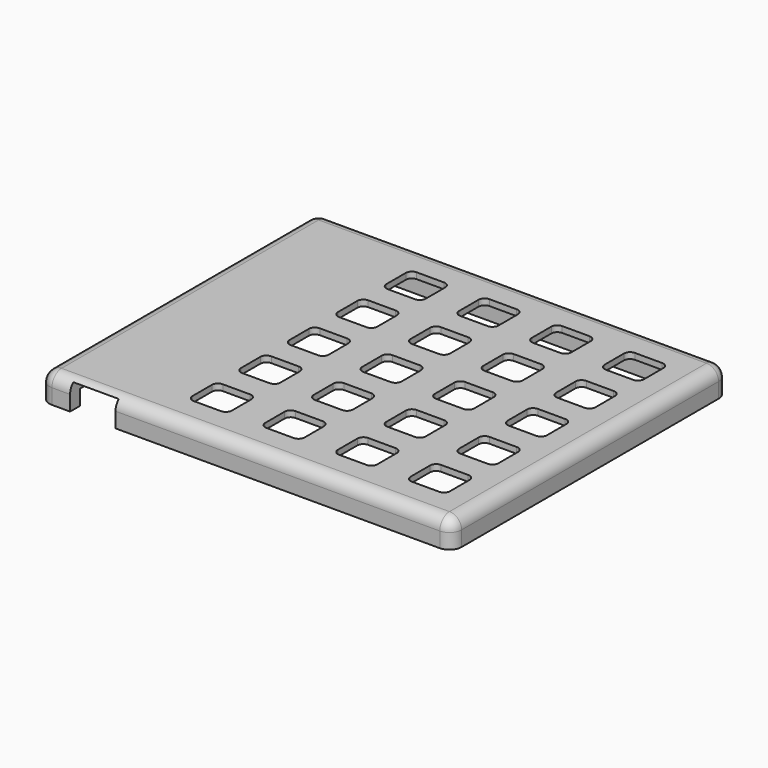
from build123d import *

# Parameters (mm, degrees)
F0_W          = 107.95
F0_H          = 90.4875
F1_DEPTH      = 7.14375
F2_W          = 101.6
F2_H          = 81.75625
F3_DEPTH      = 3.96875
F4_W          = 15.08125
F4_H          = 14.2875
F4_W_2        = 11.90625
F4_H_2        = 11.1125
F4_W_3        = 1.5875
F4_H_3        = 1.5875
F5_DEPTH      = 1.5875
F8_DEPTH      = 25.4
F9_W          = 11.90625
F9_H          = 6.35
F10_DEPTH     = 4.7625
F11_T1_DEPTH  = 101.6
F11_T3_DEPTH  = 84.1375
F11_T5_DEPTH  = 11.90625
F11_S9_W      = 3.175
F11_S9_H      = 3.175
F11_T10_DEPTH = 3.175
F11_S15_W     = 3.175
F11_S15_H     = 3.175
F11_T16_DEPTH = 3.175
F11_S21_W     = 3.175
F11_S21_H     = 3.175
F11_T22_DEPTH = 3.175
F11_S27_W     = 3.175
F11_S27_H     = 3.175
F11_T28_DEPTH = 3.175
F13_W         = 4.92252
F13_H         = 5.31749
F14_DEPTH     = 3.96875


# Not quite as in the source:
# - a fillet or chamfer that OpenCascade refuses, or shapes differently, is made with other operations: its cross-section is extruded or revolved along the edge and cut away or added


with BuildPart() as f1:
    # F0 (on Top) → F1 (new body)
    with BuildSketch(Plane.XY):
        Rectangle(F0_W, F0_H)
    extrude(amount=F1_DEPTH)

    # F2 (on face) → F3 (cut)
    with BuildSketch(Plane(origin=(0, 0, 0), x_dir=(1, 0, 0), z_dir=(0, 0, -1))):
        with Locations((0, 1.190625)):
            Rectangle(F2_W, F2_H)
    extrude(amount=-F3_DEPTH, mode=Mode.SUBTRACT)

    # F4 (on face) → F5 (cut)
    with BuildSketch(Plane(origin=(0, 0, 3.96875), x_dir=(1, 0, 0), z_dir=(0, 0, -1))):
        Polygon((-24.60625, 38.89375), (-24.60625, 34.7782671452), (-24.60625, 24.60625), (-9.525, 24.60625), (-9.525, 38.89375), align=None)
        Polygon((-23.01875, 26.19375), (-23.01875, 34.7782671452), (-23.01875, 37.30625), (-11.1125, 37.30625), (-11.1125, 26.19375), align=None, mode=Mode.SUBTRACT)
        with Locations((1.984375, 31.75)):
            Rectangle(F4_W, F4_H)
        with Locations((1.984375, 31.75)):
            Rectangle(F4_W_2, F4_H_2, mode=Mode.SUBTRACT)
        with Locations((21.034375, 31.75)):
            Rectangle(F4_W, F4_H)
        with Locations((21.034375, 31.75)):
            Rectangle(F4_W_2, F4_H_2, mode=Mode.SUBTRACT)
        with Locations((40.084375, 15.875)):
            Rectangle(F4_W, F4_H)
        with Locations((40.084375, 15.875)):
            Rectangle(F4_W_2, F4_H_2, mode=Mode.SUBTRACT)
        with Locations((21.034375, 15.875)):
            Rectangle(F4_W, F4_H)
        with Locations((21.034375, 15.875)):
            Rectangle(F4_W_2, F4_H_2, mode=Mode.SUBTRACT)
        with Locations((1.984375, 15.875)):
            Rectangle(F4_W, F4_H)
        with Locations((1.984375, 15.875)):
            Rectangle(F4_W_2, F4_H_2, mode=Mode.SUBTRACT)
        with Locations((-17.065625, 15.875)):
            Rectangle(F4_W, F4_H)
        with Locations((-17.065625, 15.875)):
            Rectangle(F4_W_2, F4_H_2, mode=Mode.SUBTRACT)
        with Locations((-17.065625, 0)):
            Rectangle(F4_W, F4_H)
        with Locations((-17.065625, 0)):
            Rectangle(F4_W_2, F4_H_2, mode=Mode.SUBTRACT)
        with Locations((1.984375, 0)):
            Rectangle(F4_W, F4_H)
        with Locations((1.984375, 0)):
            Rectangle(F4_W_2, F4_H_2, mode=Mode.SUBTRACT)
        with Locations((21.034375, 0)):
            Rectangle(F4_W, F4_H)
        with Locations((21.034375, 0)):
            Rectangle(F4_W_2, F4_H_2, mode=Mode.SUBTRACT)
        with Locations((40.084375, 0)):
            Rectangle(F4_W, F4_H)
        with Locations((40.084375, 0)):
            Rectangle(F4_W_2, F4_H_2, mode=Mode.SUBTRACT)
        with Locations((-17.065625, -15.875)):
            Rectangle(F4_W, F4_H)
        with Locations((-17.065625, -15.875)):
            Rectangle(F4_W_2, F4_H_2, mode=Mode.SUBTRACT)
        with Locations((1.984375, -15.875)):
            Rectangle(F4_W, F4_H)
        with Locations((1.984375, -15.875)):
            Rectangle(F4_W_2, F4_H_2, mode=Mode.SUBTRACT)
        with Locations((21.034375, -15.875)):
            Rectangle(F4_W, F4_H)
        with Locations((21.034375, -15.875)):
            Rectangle(F4_W_2, F4_H_2, mode=Mode.SUBTRACT)
        with Locations((40.084375, -15.875)):
            Rectangle(F4_W, F4_H)
        with Locations((40.084375, -15.875)):
            Rectangle(F4_W_2, F4_H_2, mode=Mode.SUBTRACT)
        Polygon((32.54375, -38.89375), (41.1446839571, -38.89375), (47.625, -38.89375), (47.625, -24.60625), (32.54375, -24.60625), align=None)
        Polygon((46.0375, -37.30625), (41.1446839571, -37.30625), (34.13125, -37.30625), (34.13125, -26.19375), (46.0375, -26.19375), align=None, mode=Mode.SUBTRACT)
        with Locations((21.034375, -31.75)):
            Rectangle(F4_W, F4_H)
        with Locations((21.034375, -31.75)):
            Rectangle(F4_W_2, F4_H_2, mode=Mode.SUBTRACT)
        with Locations((1.984375, -31.75)):
            Rectangle(F4_W, F4_H)
        with Locations((1.984375, -31.75)):
            Rectangle(F4_W_2, F4_H_2, mode=Mode.SUBTRACT)
        with Locations((-17.065625, -31.75)):
            Rectangle(F4_W, F4_H)
        with Locations((-17.065625, -31.75)):
            Rectangle(F4_W_2, F4_H_2, mode=Mode.SUBTRACT)
        Polygon((46.0375, 37.30625), (46.0375, 38.89375), (32.54375, 38.89375), (32.54375, 24.60625), (47.625, 24.60625), (47.625, 37.30625), align=None)
        with Locations((40.084375, 31.75)):
            Rectangle(F4_W_2, F4_H_2, mode=Mode.SUBTRACT)
        Polygon((-23.01875, 37.30625), (-23.01875, 34.7782671452), (-23.01875, 26.19375), (-11.1125, 26.19375), (-11.1125, 37.30625), align=None)
        with Locations((1.984375, 31.75)):
            Rectangle(F4_W_2, F4_H_2)
        with Locations((21.034375, 31.75)):
            Rectangle(F4_W_2, F4_H_2)
        with Locations((40.084375, 31.75)):
            Rectangle(F4_W_2, F4_H_2)
        with Locations((40.084375, 15.875)):
            Rectangle(F4_W_2, F4_H_2)
        with Locations((21.034375, 15.875)):
            Rectangle(F4_W_2, F4_H_2)
        with Locations((1.984375, 15.875)):
            Rectangle(F4_W_2, F4_H_2)
        with Locations((-17.065625, 15.875)):
            Rectangle(F4_W_2, F4_H_2)
        with Locations((-17.065625, 0)):
            Rectangle(F4_W_2, F4_H_2)
        with Locations((1.984375, 0)):
            Rectangle(F4_W_2, F4_H_2)
        with Locations((21.034375, 0)):
            Rectangle(F4_W_2, F4_H_2)
        with Locations((40.084375, 0)):
            Rectangle(F4_W_2, F4_H_2)
        with Locations((-17.065625, -15.875)):
            Rectangle(F4_W_2, F4_H_2)
        with Locations((1.984375, -15.875)):
            Rectangle(F4_W_2, F4_H_2)
        with Locations((21.034375, -15.875)):
            Rectangle(F4_W_2, F4_H_2)
        with Locations((40.084375, -15.875)):
            Rectangle(F4_W_2, F4_H_2)
        Polygon((34.13125, -37.30625), (41.1446839571, -37.30625), (46.0375, -37.30625), (46.0375, -26.19375), (34.13125, -26.19375), align=None)
        with Locations((21.034375, -31.75)):
            Rectangle(F4_W_2, F4_H_2)
        with Locations((1.984375, -31.75)):
            Rectangle(F4_W_2, F4_H_2)
        with Locations((-17.065625, -31.75)):
            Rectangle(F4_W_2, F4_H_2)
        with Locations((46.83125, 38.1)):
            Rectangle(F4_W_3, F4_H_3)
    extrude(amount=-F5_DEPTH, mode=Mode.SUBTRACT)

    # F7 (on face) → F8 (cut)
    with BuildSketch(Plane.XY.offset(7.14375)):
        with BuildLine():
            Line((43.65625, -26.9875), (36.5125, -26.9875))
            ThreePointArc((36.5125, -26.9875), (35.3899679849, -27.4524679849), (34.925, -28.575))
            Line((34.925, -28.575), (34.925, -34.925))
            ThreePointArc((34.925, -34.925), (35.3899679849, -36.0475320151), (36.5125, -36.5125))
            Line((36.5125, -36.5125), (43.65625, -36.5125))
            ThreePointArc((43.65625, -36.5125), (44.7787820151, -36.0475320151), (45.24375, -34.925))
            Line((45.24375, -34.925), (45.24375, -28.575))
            ThreePointArc((45.24375, -28.575), (44.7787820151, -27.4524679849), (43.65625, -26.9875))
        make_face()
        with BuildLine():
            Line((43.65625, -11.1125), (36.5125, -11.1125))
            ThreePointArc((36.5125, -11.1125), (35.3899679849, -11.5774679849), (34.925, -12.7))
            Line((34.925, -12.7), (34.925, -19.05))
            ThreePointArc((34.925, -19.05), (35.3899679849, -20.1725320151), (36.5125, -20.6375))
            Line((36.5125, -20.6375), (43.65625, -20.6375))
            ThreePointArc((43.65625, -20.6375), (44.7787820151, -20.1725320151), (45.24375, -19.05))
            Line((45.24375, -19.05), (45.24375, -12.7))
            ThreePointArc((45.24375, -12.7), (44.7787820151, -11.5774679849), (43.65625, -11.1125))
        make_face()
        with BuildLine():
            Line((24.60625, -11.1125), (17.4625, -11.1125))
            ThreePointArc((17.4625, -11.1125), (16.3399679849, -11.5774679849), (15.875, -12.7))
            Line((15.875, -12.7), (15.875, -19.05))
            ThreePointArc((15.875, -19.05), (16.3399679849, -20.1725320151), (17.4625, -20.6375))
            Line((17.4625, -20.6375), (24.60625, -20.6375))
            ThreePointArc((24.60625, -20.6375), (25.7287820151, -20.1725320151), (26.19375, -19.05))
            Line((26.19375, -19.05), (26.19375, -12.7))
            ThreePointArc((26.19375, -12.7), (25.7287820151, -11.5774679849), (24.60625, -11.1125))
        make_face()
        with BuildLine():
            Line((24.60625, -26.9875), (17.4625, -26.9875))
            ThreePointArc((17.4625, -26.9875), (16.3399679849, -27.4524679849), (15.875, -28.575))
            Line((15.875, -28.575), (15.875, -34.925))
            ThreePointArc((15.875, -34.925), (16.3399679849, -36.0475320151), (17.4625, -36.5125))
            Line((17.4625, -36.5125), (24.60625, -36.5125))
            ThreePointArc((24.60625, -36.5125), (25.7287820151, -36.0475320151), (26.19375, -34.925))
            Line((26.19375, -34.925), (26.19375, -28.575))
            ThreePointArc((26.19375, -28.575), (25.7287820151, -27.4524679849), (24.60625, -26.9875))
        make_face()
        with BuildLine():
            Line((5.55625, -26.9875), (-1.5875, -26.9875))
            ThreePointArc((-1.5875, -26.9875), (-2.7100320151, -27.4524679849), (-3.175, -28.575))
            Line((-3.175, -28.575), (-3.175, -34.925))
            ThreePointArc((-3.175, -34.925), (-2.7100320151, -36.0475320151), (-1.5875, -36.5125))
            Line((-1.5875, -36.5125), (5.55625, -36.5125))
            ThreePointArc((5.55625, -36.5125), (6.6787820151, -36.0475320151), (7.14375, -34.925))
            Line((7.14375, -34.925), (7.14375, -28.575))
            ThreePointArc((7.14375, -28.575), (6.6787820151, -27.4524679849), (5.55625, -26.9875))
        make_face()
        with BuildLine():
            Line((5.55625, -11.1125), (-1.5875, -11.1125))
            ThreePointArc((-1.5875, -11.1125), (-2.7100320151, -11.5774679849), (-3.175, -12.7))
            Line((-3.175, -12.7), (-3.175, -19.05))
            ThreePointArc((-3.175, -19.05), (-2.7100320151, -20.1725320151), (-1.5875, -20.6375))
            Line((-1.5875, -20.6375), (5.55625, -20.6375))
            ThreePointArc((5.55625, -20.6375), (6.6787820151, -20.1725320151), (7.14375, -19.05))
            Line((7.14375, -19.05), (7.14375, -12.7))
            ThreePointArc((7.14375, -12.7), (6.6787820151, -11.5774679849), (5.55625, -11.1125))
        make_face()
        with BuildLine():
            Line((-13.49375, -11.1125), (-20.6375, -11.1125))
            ThreePointArc((-20.6375, -11.1125), (-21.7600320151, -11.5774679849), (-22.225, -12.7))
            Line((-22.225, -12.7), (-22.225, -19.05))
            ThreePointArc((-22.225, -19.05), (-21.7600320151, -20.1725320151), (-20.6375, -20.6375))
            Line((-20.6375, -20.6375), (-13.49375, -20.6375))
            ThreePointArc((-13.49375, -20.6375), (-12.3712179849, -20.1725320151), (-11.90625, -19.05))
            Line((-11.90625, -19.05), (-11.90625, -12.7))
            ThreePointArc((-11.90625, -12.7), (-12.3712179849, -11.5774679849), (-13.49375, -11.1125))
        make_face()
        with BuildLine():
            Line((-13.49375, -26.9875), (-20.6375, -26.9875))
            ThreePointArc((-20.6375, -26.9875), (-21.7600320151, -27.4524679849), (-22.225, -28.575))
            Line((-22.225, -28.575), (-22.225, -34.925))
            ThreePointArc((-22.225, -34.925), (-21.7600320151, -36.0475320151), (-20.6375, -36.5125))
            Line((-20.6375, -36.5125), (-13.49375, -36.5125))
            ThreePointArc((-13.49375, -36.5125), (-12.3712179849, -36.0475320151), (-11.90625, -34.925))
            Line((-11.90625, -34.925), (-11.90625, -28.575))
            ThreePointArc((-11.90625, -28.575), (-12.3712179849, -27.4524679849), (-13.49375, -26.9875))
        make_face()
        with BuildLine():
            Line((-13.49375, 4.7625), (-20.6375, 4.7625))
            ThreePointArc((-20.6375, 4.7625), (-21.7600320151, 4.2975320151), (-22.225, 3.175))
            Line((-22.225, 3.175), (-22.225, -3.175))
            ThreePointArc((-22.225, -3.175), (-21.7600320151, -4.2975320151), (-20.6375, -4.7625))
            Line((-20.6375, -4.7625), (-13.49375, -4.7625))
            ThreePointArc((-13.49375, -4.7625), (-12.3712179849, -4.2975320151), (-11.90625, -3.175))
            Line((-11.90625, -3.175), (-11.90625, 3.175))
            ThreePointArc((-11.90625, 3.175), (-12.3712179849, 4.2975320151), (-13.49375, 4.7625))
        make_face()
        with BuildLine():
            Line((-13.49375, 20.6375), (-20.6375, 20.6375))
            ThreePointArc((-20.6375, 20.6375), (-21.7600320151, 20.1725320151), (-22.225, 19.05))
            Line((-22.225, 19.05), (-22.225, 12.7))
            ThreePointArc((-22.225, 12.7), (-21.7600320151, 11.5774679849), (-20.6375, 11.1125))
            Line((-20.6375, 11.1125), (-13.49375, 11.1125))
            ThreePointArc((-13.49375, 11.1125), (-12.3712179849, 11.5774679849), (-11.90625, 12.7))
            Line((-11.90625, 12.7), (-11.90625, 19.05))
            ThreePointArc((-11.90625, 19.05), (-12.3712179849, 20.1725320151), (-13.49375, 20.6375))
        make_face()
        with BuildLine():
            Line((-13.49375, 36.5125), (-20.6375, 36.5125))
            ThreePointArc((-20.6375, 36.5125), (-21.7600320151, 36.0475320151), (-22.225, 34.925))
            Line((-22.225, 34.925), (-22.225, 28.575))
            ThreePointArc((-22.225, 28.575), (-21.7600320151, 27.4524679849), (-20.6375, 26.9875))
            Line((-20.6375, 26.9875), (-13.49375, 26.9875))
            ThreePointArc((-13.49375, 26.9875), (-12.3712179849, 27.4524679849), (-11.90625, 28.575))
            Line((-11.90625, 28.575), (-11.90625, 34.925))
            ThreePointArc((-11.90625, 34.925), (-12.3712179849, 36.0475320151), (-13.49375, 36.5125))
        make_face()
        with BuildLine():
            Line((5.55625, 36.5125), (-1.5875, 36.5125))
            ThreePointArc((-1.5875, 36.5125), (-2.7100320151, 36.0475320151), (-3.175, 34.925))
            Line((-3.175, 34.925), (-3.175, 28.575))
            ThreePointArc((-3.175, 28.575), (-2.7100320151, 27.4524679849), (-1.5875, 26.9875))
            Line((-1.5875, 26.9875), (5.55625, 26.9875))
            ThreePointArc((5.55625, 26.9875), (6.6787820151, 27.4524679849), (7.14375, 28.575))
            Line((7.14375, 28.575), (7.14375, 34.925))
            ThreePointArc((7.14375, 34.925), (6.6787820151, 36.0475320151), (5.55625, 36.5125))
        make_face()
        with BuildLine():
            Line((24.60625, 36.5125), (17.4625, 36.5125))
            ThreePointArc((17.4625, 36.5125), (16.3399679849, 36.0475320151), (15.875, 34.925))
            Line((15.875, 34.925), (15.875, 28.575))
            ThreePointArc((15.875, 28.575), (16.3399679849, 27.4524679849), (17.4625, 26.9875))
            Line((17.4625, 26.9875), (24.60625, 26.9875))
            ThreePointArc((24.60625, 26.9875), (25.7287820151, 27.4524679849), (26.19375, 28.575))
            Line((26.19375, 28.575), (26.19375, 34.925))
            ThreePointArc((26.19375, 34.925), (25.7287820151, 36.0475320151), (24.60625, 36.5125))
        make_face()
        with BuildLine():
            Line((43.65625, 36.5125), (36.5125, 36.5125))
            ThreePointArc((36.5125, 36.5125), (35.3899679849, 36.0475320151), (34.925, 34.925))
            Line((34.925, 34.925), (34.925, 28.575))
            ThreePointArc((34.925, 28.575), (35.3899679849, 27.4524679849), (36.5125, 26.9875))
            Line((36.5125, 26.9875), (43.65625, 26.9875))
            ThreePointArc((43.65625, 26.9875), (44.7787820151, 27.4524679849), (45.24375, 28.575))
            Line((45.24375, 28.575), (45.24375, 34.925))
            ThreePointArc((45.24375, 34.925), (44.7787820151, 36.0475320151), (43.65625, 36.5125))
        make_face()
        with BuildLine():
            Line((43.65625, 20.6375), (36.5125, 20.6375))
            ThreePointArc((36.5125, 20.6375), (35.3899679849, 20.1725320151), (34.925, 19.05))
            Line((34.925, 19.05), (34.925, 12.7))
            ThreePointArc((34.925, 12.7), (35.3899679849, 11.5774679849), (36.5125, 11.1125))
            Line((36.5125, 11.1125), (43.65625, 11.1125))
            ThreePointArc((43.65625, 11.1125), (44.7787820151, 11.5774679849), (45.24375, 12.7))
            Line((45.24375, 12.7), (45.24375, 19.05))
            ThreePointArc((45.24375, 19.05), (44.7787820151, 20.1725320151), (43.65625, 20.6375))
        make_face()
        with BuildLine():
            Line((43.65625, 4.7625), (36.5125, 4.7625))
            ThreePointArc((36.5125, 4.7625), (35.3899679849, 4.2975320151), (34.925, 3.175))
            Line((34.925, 3.175), (34.925, -3.175))
            ThreePointArc((34.925, -3.175), (35.3899679849, -4.2975320151), (36.5125, -4.7625))
            Line((36.5125, -4.7625), (43.65625, -4.7625))
            ThreePointArc((43.65625, -4.7625), (44.7787820151, -4.2975320151), (45.24375, -3.175))
            Line((45.24375, -3.175), (45.24375, 3.175))
            ThreePointArc((45.24375, 3.175), (44.7787820151, 4.2975320151), (43.65625, 4.7625))
        make_face()
        with BuildLine():
            Line((24.60625, 4.7625), (17.4625, 4.7625))
            ThreePointArc((17.4625, 4.7625), (16.3399679849, 4.2975320151), (15.875, 3.175))
            Line((15.875, 3.175), (15.875, -3.175))
            ThreePointArc((15.875, -3.175), (16.3399679849, -4.2975320151), (17.4625, -4.7625))
            Line((17.4625, -4.7625), (24.60625, -4.7625))
            ThreePointArc((24.60625, -4.7625), (25.7287820151, -4.2975320151), (26.19375, -3.175))
            Line((26.19375, -3.175), (26.19375, 3.175))
            ThreePointArc((26.19375, 3.175), (25.7287820151, 4.2975320151), (24.60625, 4.7625))
        make_face()
        with BuildLine():
            Line((5.55625, 4.7625), (-1.5875, 4.7625))
            ThreePointArc((-1.5875, 4.7625), (-2.7100320151, 4.2975320151), (-3.175, 3.175))
            Line((-3.175, 3.175), (-3.175, -3.175))
            ThreePointArc((-3.175, -3.175), (-2.7100320151, -4.2975320151), (-1.5875, -4.7625))
            Line((-1.5875, -4.7625), (5.55625, -4.7625))
            ThreePointArc((5.55625, -4.7625), (6.6787820151, -4.2975320151), (7.14375, -3.175))
            Line((7.14375, -3.175), (7.14375, 3.175))
            ThreePointArc((7.14375, 3.175), (6.6787820151, 4.2975320151), (5.55625, 4.7625))
        make_face()
        with BuildLine():
            Line((5.55625, 20.6375), (-1.5875, 20.6375))
            ThreePointArc((-1.5875, 20.6375), (-2.7100320151, 20.1725320151), (-3.175, 19.05))
            Line((-3.175, 19.05), (-3.175, 12.7))
            ThreePointArc((-3.175, 12.7), (-2.7100320151, 11.5774679849), (-1.5875, 11.1125))
            Line((-1.5875, 11.1125), (5.55625, 11.1125))
            ThreePointArc((5.55625, 11.1125), (6.6787820151, 11.5774679849), (7.14375, 12.7))
            Line((7.14375, 12.7), (7.14375, 19.05))
            ThreePointArc((7.14375, 19.05), (6.6787820151, 20.1725320151), (5.55625, 20.6375))
        make_face()
        with BuildLine():
            Line((24.60625, 20.6375), (17.4625, 20.6375))
            ThreePointArc((17.4625, 20.6375), (16.3399679849, 20.1725320151), (15.875, 19.05))
            Line((15.875, 19.05), (15.875, 12.7))
            ThreePointArc((15.875, 12.7), (16.3399679849, 11.5774679849), (17.4625, 11.1125))
            Line((17.4625, 11.1125), (24.60625, 11.1125))
            ThreePointArc((24.60625, 11.1125), (25.7287820151, 11.5774679849), (26.19375, 12.7))
            Line((26.19375, 12.7), (26.19375, 19.05))
            ThreePointArc((26.19375, 19.05), (25.7287820151, 20.1725320151), (24.60625, 20.6375))
        make_face()
    extrude(amount=-F8_DEPTH, mode=Mode.SUBTRACT)

    # F9 (on face) → F10 (cut)
    with BuildSketch(Plane.XZ.offset(45.24375)):
        with Locations((-40.084375, 3.175)):
            Rectangle(F9_W, F9_H)
    extrude(amount=-F10_DEPTH, mode=Mode.SUBTRACT)

    # F11: fillet of radius 3.175 on 8 edges, made by hand

    # F11_s2 → F11_t1 (cut)
    with BuildSketch(Plane.YZ.offset(-50.8)):
        with BuildLine():
            ThreePointArc((-45.24375, 3.96875), (-44.3138140303, 6.2138140303), (-42.06875, 7.14375))
            Line((-42.06875, 7.14375), (-45.24375, 7.14375))
            Line((-45.24375, 7.14375), (-45.24375, 3.96875))
        make_face()
        with BuildLine():
            ThreePointArc((42.06875, 7.14375), (44.3138140303, 6.2138140303), (45.24375, 3.96875))
            Line((45.24375, 3.96875), (45.24375, 7.14375))
            Line((45.24375, 7.14375), (42.06875, 7.14375))
        make_face()
    extrude(amount=F11_T1_DEPTH, mode=Mode.SUBTRACT)

    # F11_s4 → F11_t3 (cut)
    with BuildSketch(Plane.XZ.offset(-42.06875)):
        with BuildLine():
            ThreePointArc((-50.8, 7.14375), (-53.0450640303, 6.2138140303), (-53.975, 3.96875))
            Line((-53.975, 3.96875), (-53.975, 7.14375))
            Line((-53.975, 7.14375), (-50.8, 7.14375))
        make_face()
        with BuildLine():
            ThreePointArc((53.975, 3.96875), (53.0450640303, 6.2138140303), (50.8, 7.14375))
            Line((50.8, 7.14375), (53.975, 7.14375))
            Line((53.975, 7.14375), (53.975, 3.96875))
        make_face()
    extrude(amount=F11_T3_DEPTH, mode=Mode.SUBTRACT)

    # F11_s6 → F11_t5 (cut)
    with BuildSketch(Plane.XY.offset(-7.9375)):
        with BuildLine():
            ThreePointArc((-53.975, 42.06875), (-53.0450640303, 44.3138140303), (-50.8, 45.24375))
            Line((-50.8, 45.24375), (-53.975, 45.24375))
            Line((-53.975, 45.24375), (-53.975, 42.06875))
        make_face()
        with BuildLine():
            ThreePointArc((-50.8, -45.24375), (-53.0450640303, -44.3138140303), (-53.975, -42.06875))
            Line((-53.975, -42.06875), (-53.975, -45.24375))
            Line((-53.975, -45.24375), (-50.8, -45.24375))
        make_face()
        with BuildLine():
            ThreePointArc((50.8, -45.24375), (53.0450640303, -44.3138140303), (53.975, -42.06875))
            Line((53.975, -42.06875), (53.975, -45.24375))
            Line((53.975, -45.24375), (50.8, -45.24375))
        make_face()
        with BuildLine():
            ThreePointArc((53.975, 42.06875), (53.0450640303, 44.3138140303), (50.8, 45.24375))
            Line((50.8, 45.24375), (53.975, 45.24375))
            Line((53.975, 45.24375), (53.975, 42.06875))
        make_face()
    extrude(amount=F11_T5_DEPTH, mode=Mode.SUBTRACT)


with BuildPart() as f11_tool8:
    # F11_s9 → F11_t10 (new body)
    with BuildSketch(Plane.XZ.offset(42.06875)):
        with Locations((-52.3875, 5.55625)):
            Rectangle(F11_S9_W, F11_S9_H)
    extrude(amount=F11_T10_DEPTH)

    # F11_s11 → F11_t12 (revolve, cut)
    with BuildSketch(Plane(origin=(-50.8, -42.06875, 3.96875), x_dir=(0.7071067812, 0, -0.7071067812), z_dir=(-0.7071067812, 0, -0.7071067812))):
        with BuildLine():
            ThreePointArc((0, -3.175), (3.175, 0), (0, 3.175))
            Line((0, 3.175), (0, -3.175))
        make_face()
    revolve(axis=Axis((-50.8, -42.06875, 3.96875), (0, -1, 0)), mode=Mode.SUBTRACT)


with BuildPart() as f1_1:
    add(f1.part)

    # F11_t7: cut F11_tool8
    add(f11_tool8.part, mode=Mode.SUBTRACT)


with BuildPart() as f11_tool14:
    # F11_s15 → F11_t16 (new body)
    with BuildSketch(Plane.XZ.offset(42.06875)):
        with Locations((52.3875, 5.55625)):
            Rectangle(F11_S15_W, F11_S15_H)
    extrude(amount=F11_T16_DEPTH)

    # F11_s17 → F11_t18 (revolve, cut)
    with BuildSketch(Plane(origin=(50.8, -42.06875, 3.96875), x_dir=(-0.7071067812, 0, -0.7071067812), z_dir=(-0.7071067812, 0, 0.7071067812))):
        with BuildLine():
            ThreePointArc((0, -3.175), (3.175, 0), (0, 3.175))
            Line((0, 3.175), (0, -3.175))
        make_face()
    revolve(axis=Axis((50.8, -42.06875, 3.96875), (0, -1, 0)), mode=Mode.SUBTRACT)


with BuildPart() as f1_2:
    add(f1_1.part)

    # F11_t13: cut F11_tool14
    add(f11_tool14.part, mode=Mode.SUBTRACT)


with BuildPart() as f11_tool20:
    # F11_s21 → F11_t22 (new body)
    with BuildSketch(Plane.XZ.offset(-42.06875)):
        with Locations((-52.3875, 5.55625)):
            Rectangle(F11_S21_W, F11_S21_H)
    extrude(amount=-F11_T22_DEPTH)

    # F11_s23 → F11_t24 (revolve, cut)
    with BuildSketch(Plane(origin=(-50.8, 42.06875, 3.96875), x_dir=(0.7071067812, 0, -0.7071067812), z_dir=(0.7071067812, 0, 0.7071067812))):
        with BuildLine():
            ThreePointArc((0, -3.175), (3.175, 0), (0, 3.175))
            Line((0, 3.175), (0, -3.175))
        make_face()
    revolve(axis=Axis((-50.8, 42.06875, 3.96875), (0, 1, 0)), mode=Mode.SUBTRACT)


with BuildPart() as f1_3:
    add(f1_2.part)

    # F11_t19: cut F11_tool20
    add(f11_tool20.part, mode=Mode.SUBTRACT)


with BuildPart() as f11_tool26:
    # F11_s27 → F11_t28 (new body)
    with BuildSketch(Plane.XZ.offset(-42.06875)):
        with Locations((52.3875, 5.55625)):
            Rectangle(F11_S27_W, F11_S27_H)
    extrude(amount=-F11_T28_DEPTH)

    # F11_s29 → F11_t30 (revolve, cut)
    with BuildSketch(Plane(origin=(50.8, 42.06875, 3.96875), x_dir=(-0.7071067812, 0, -0.7071067812), z_dir=(0.7071067812, 0, -0.7071067812))):
        with BuildLine():
            ThreePointArc((0, -3.175), (3.175, 0), (0, 3.175))
            Line((0, 3.175), (0, -3.175))
        make_face()
    revolve(axis=Axis((50.8, 42.06875, 3.96875), (0, 1, 0)), mode=Mode.SUBTRACT)


with BuildPart() as f1_4:
    add(f1_3.part)

    # F11_t25: cut F11_tool26
    add(f11_tool26.part, mode=Mode.SUBTRACT)

    # F13 (on face) → F14 (join)
    with BuildSketch(Plane(origin=(0, 0, 0), x_dir=(1, 0, 0), z_dir=(0, 0, -1))):
        Polygon((47.625, 34.37001), (50.8, 34.37001), (50.8, 42.06875), (47.625, 42.06875), (47.625, 38.89375), align=None)
        with Locations((-48.33874, -37.028755)):
            Rectangle(F13_W, F13_H)
        Polygon((47.625, -38.89375), (47.625, -39.6875), (48.81626, -39.6875), (50.8, -39.6875), (50.8, -36.91001), (50.8, -34.37001), (47.625, -34.37001), align=None)
    extrude(amount=-F14_DEPTH)


solid = f1_4.part
